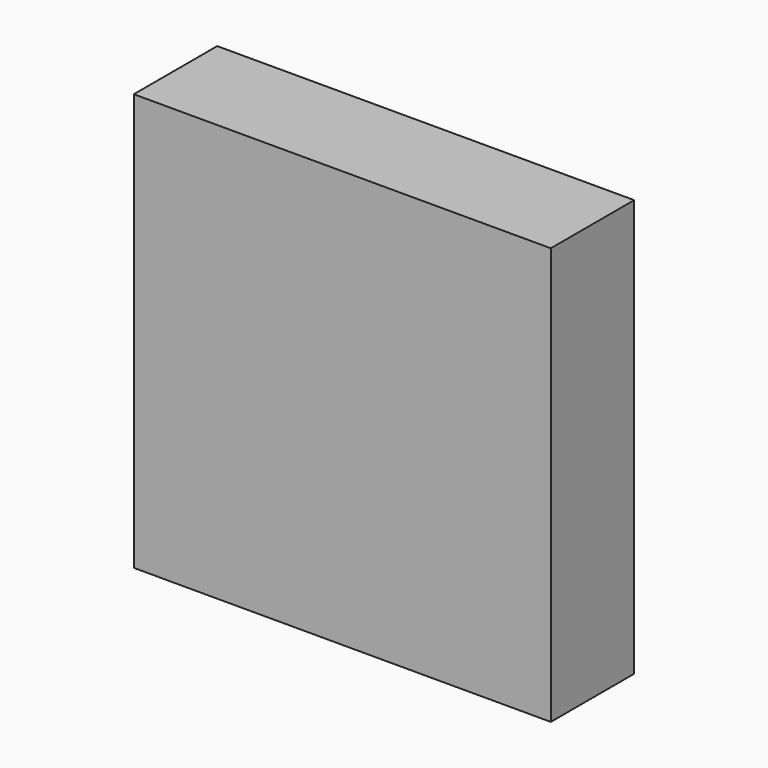
from build123d import *

# Parameters (mm, degrees)
F0_W     = 80
F0_H     = 80
F1_DEPTH = 20
F3_D     = 8
F3_DEPTH = 15
F3_TIP   = 2.4034424761
F4_DEPTH = 10
F5_DEPTH = 15


with BuildPart() as f1:
    # F0 (on Front) → F1 (new body)
    with BuildSketch(Plane.XZ):
        Rectangle(F0_W, F0_H)
    extrude(amount=F1_DEPTH)

    # F3
    with Locations(Plane(origin=(0, 0, 0), x_dir=(-1, 0, 0), z_dir=(0, 1, 0))):
        with Locations((-25, -32), (15, -32)):
            Hole(F3_D / 2, depth=F3_DEPTH)
            with Locations((0, 0, -(F3_DEPTH + F3_TIP / 2))):  # 118° drill point
                Cone(0, F3_D / 2, F3_TIP, mode=Mode.SUBTRACT)

    # F2 (on face) → F4 (cut)
    with BuildSketch(Plane(origin=(0, 0, 0), x_dir=(-1, 0, 0), z_dir=(0, 1, 0))):
        with BuildLine():
            ThreePointArc((-35, -15), (-32.0710678119, -22.0710678119), (-25, -25))
            Line((-25, -25), (15, -25))
            ThreePointArc((15, -25), (22.0710678119, -22.0710678119), (25, -15))
            Line((25, -15), (25, 25))
            ThreePointArc((25, 25), (22.0710678119, 32.0710678119), (15, 35))
            Line((15, 35), (-25, 35))
            ThreePointArc((-25, 35), (-32.0710678119, 32.0710678119), (-35, 25))
            Line((-35, 25), (-35, -15))
        make_face()
        with BuildLine():
            ThreePointArc((-24.4594421512, 19), (-22.7020828383, 23.2426406871), (-18.4594421512, 25))
            Line((-18.4594421512, 25), (9.5405578488, 25))
            ThreePointArc((9.5405578488, 25), (13.7831985359, 23.2426406871), (15.5405578488, 19))
            Line((15.5405578488, 19), (15.5405578488, -9))
            ThreePointArc((15.5405578488, -9), (13.7831985359, -13.2426406871), (9.5405578488, -15))
            Line((9.5405578488, -15), (-18.4594421512, -15))
            ThreePointArc((-18.4594421512, -15), (-22.7020828383, -13.2426406871), (-24.4594421512, -9))
            Line((-24.4594421512, -9), (-24.4594421512, 19))
        make_face(mode=Mode.SUBTRACT)
    extrude(amount=-F4_DEPTH, mode=Mode.SUBTRACT)

    # F2 (on face) → F5 (cut)
    with BuildSketch(Plane(origin=(0, 0, 0), x_dir=(-1, 0, 0), z_dir=(0, 1, 0))):
        with BuildLine():
            Line((9.5405578488, 25), (-18.4594421512, 25))
            ThreePointArc((-18.4594421512, 25), (-22.7020828383, 23.2426406871), (-24.4594421512, 19))
            Line((-24.4594421512, 19), (-24.4594421512, -9))
            ThreePointArc((-24.4594421512, -9), (-22.7020828383, -13.2426406871), (-18.4594421512, -15))
            Line((-18.4594421512, -15), (9.5405578488, -15))
            ThreePointArc((9.5405578488, -15), (13.7831985359, -13.2426406871), (15.5405578488, -9))
            Line((15.5405578488, -9), (15.5405578488, 19))
            ThreePointArc((15.5405578488, 19), (13.7831985359, 23.2426406871), (9.5405578488, 25))
        make_face()
    extrude(amount=-F5_DEPTH, mode=Mode.SUBTRACT)


solid = f1.part
